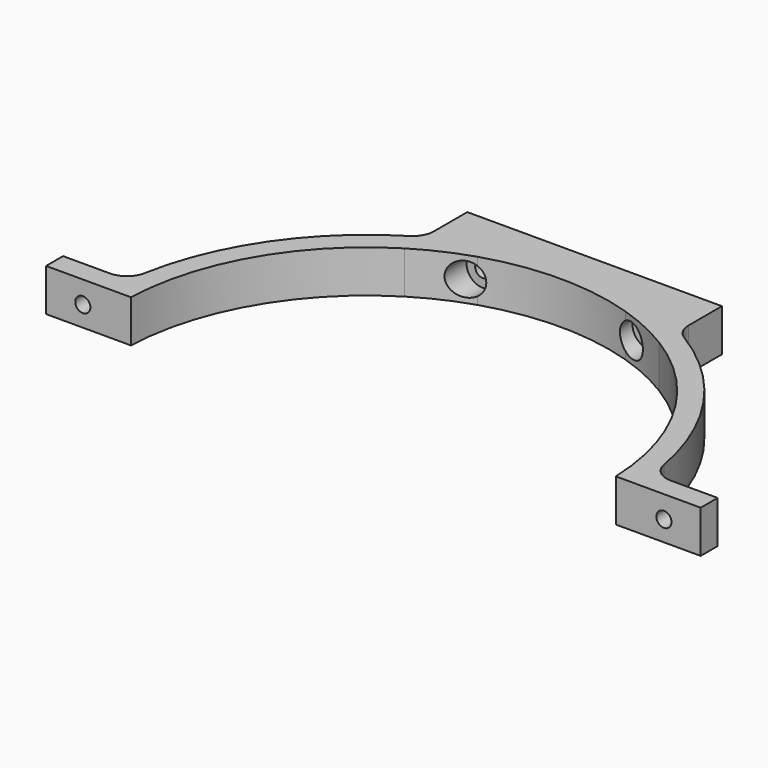
from build123d import *
from build123d import SkipClean  # not in build123d's __all__

# Parameters (mm, degrees)
F1_DEPTH       = 10
F3_D           = 3.556
F3_CBORE_D     = 7.62
F3_CBORE_DEPTH = 10
F4_DEPTH       = 10.0010001
F6_D           = 3.556
F7_R           = 5


with BuildPart() as f1:
    # F0 (on Top) → F1 (new body)
    with BuildSketch(Plane.XY):
        with BuildLine():
            ThreePointArc((30, 48.6428052234), (49.4079280032, 28.7224502859), (57.1149936532, 2))
            Line((57.1149936532, 2), (57.1149936532, 7))
            Line((57.1149936532, 7), (61.7545342465, 7))
            ThreePointArc((61.7545342465, 7), (51.6442091706, 34.5759766187), (30, 54.4299779533))
            Line((30, 54.4299779533), (30, 48.6428052234))
        make_face()
        with BuildLine():
            ThreePointArc((17.4212513902, 54.4299779533), (23.8865362266, 51.9187431194), (30, 48.6428052234))
            Line((30, 48.6428052234), (30, 54.4299779533))
            Line((30, 54.4299779533), (17.4212513902, 54.4299779533))
        make_face()
        with BuildLine():
            ThreePointArc((-17.4212513902, 54.4299779533), (0, 57.15), (17.4212513902, 54.4299779533))
            Line((17.4212513902, 54.4299779533), (30, 54.4299779533))
            ThreePointArc((30, 54.4299779533), (15.4886954339, 60.1890589207), (7.62e-08, 62.15))
            ThreePointArc((7.62e-08, 62.15), (-15.4886953601, 60.1890589397), (-30, 54.4299779533))
            Line((-30, 54.4299779533), (-17.4212513902, 54.4299779533))
        make_face()
        with BuildLine():
            Line((-30, 54.4299779533), (-30, 48.6428052234))
            ThreePointArc((-30, 48.6428052234), (-23.8865362266, 51.9187431194), (-17.4212513902, 54.4299779533))
            Line((-17.4212513902, 54.4299779533), (-30, 54.4299779533))
        make_face()
        with BuildLine():
            ThreePointArc((-57.1149936532, 2), (-49.4079280032, 28.7224502859), (-30, 48.6428052234))
            Line((-30, 48.6428052234), (-30, 54.4299779533))
            ThreePointArc((-30, 54.4299779533), (-51.6442091706, 34.5759766187), (-61.7545342465, 7))
            Line((-61.7545342465, 7), (-57.1149936532, 7))
            Line((-57.1149936532, 7), (-57.1149936532, 2))
        make_face()
        with BuildLine():
            Line((-77.1149936532, 2), (-62.1178114553, 2))
            ThreePointArc((-62.1178114553, 2), (-61.9866074843, 4.5036643506), (-61.7545342465, 7))
            Line((-61.7545342465, 7), (-77.1149936532, 7))
            Line((-77.1149936532, 7), (-77.1149936532, 2))
        make_face()
        with BuildLine():
            Line((-62.1178114553, 2), (-57.1149936532, 2))
            Line((-57.1149936532, 2), (-57.1149936532, 7))
            Line((-57.1149936532, 7), (-61.7545342465, 7))
            ThreePointArc((-61.7545342465, 7), (-61.9866074843, 4.5036643506), (-62.1178114553, 2))
        make_face()
        with BuildLine():
            Line((57.1149936532, 7), (57.1149936532, 2))
            Line((57.1149936532, 2), (62.1178114553, 2))
            ThreePointArc((62.1178114553, 2), (61.9866074843, 4.5036643506), (61.7545342465, 7))
            Line((61.7545342465, 7), (57.1149936532, 7))
        make_face()
        with BuildLine():
            ThreePointArc((61.7545342465, 7), (61.9866074843, 4.5036643506), (62.1178114553, 2))
            Line((62.1178114553, 2), (77.1149936532, 2))
            Line((77.1149936532, 2), (77.1149936532, 7))
            Line((77.1149936532, 7), (61.7545342465, 7))
        make_face()
        with BuildLine():
            Line((-30, 62.15), (-30, 54.4299779533))
            ThreePointArc((-30, 54.4299779533), (-15.4886953601, 60.1890589397), (7.62e-08, 62.15))
            Line((7.62e-08, 62.15), (-30, 62.15))
        make_face()
        with BuildLine():
            ThreePointArc((7.62e-08, 62.15), (15.4886954339, 60.1890589207), (30, 54.4299779533))
            Line((30, 54.4299779533), (30, 62.15))
            Line((30, 62.15), (7.62e-08, 62.15))
        make_face()
        with BuildLine():
            Line((-30, 48.6428052234), (30, 48.6428052234))
            ThreePointArc((30, 48.6428052234), (23.8865362266, 51.9187431194), (17.4212513902, 54.4299779533))
            Line((17.4212513902, 54.4299779533), (-17.4212513902, 54.4299779533))
            ThreePointArc((-17.4212513902, 54.4299779533), (-23.8865362266, 51.9187431194), (-30, 48.6428052234))
        make_face()
        Polygon((-30, 62.15), (7.62e-08, 62.15), (30, 62.15), (30, 67.15), (-30, 67.15), align=None)
    extrude(amount=F1_DEPTH)

    # F3 (through all)
    with Locations(Plane.XZ.offset(-48.6428052234)):
        with Locations((-19.558, 4.9517820589), (19.558, 4.9517820589)):
            CounterBoreHole(F3_D / 2, F3_CBORE_D / 2, F3_CBORE_DEPTH)

    # F0 (on Top) → F4 (cut, through all)
    with BuildSketch(Plane.XY):
        with BuildLine():
            Line((-30, 48.6428052234), (30, 48.6428052234))
            ThreePointArc((30, 48.6428052234), (23.8865362266, 51.9187431194), (17.4212513902, 54.4299779533))
            Line((17.4212513902, 54.4299779533), (-17.4212513902, 54.4299779533))
            ThreePointArc((-17.4212513902, 54.4299779533), (-23.8865362266, 51.9187431194), (-30, 48.6428052234))
        make_face()
    with SkipClean():  # cleaning this boolean's faces spoils the solid; the shape is the same uncleaned
        extrude(amount=F4_DEPTH, mode=Mode.SUBTRACT)

    # F6 (through all)
    with Locations(Plane.XZ.offset(-2)):
        with Locations((-68.453, 4.78035165), (68.453, 4.78035165)):
            Hole(F6_D / 2)

    # F7
    f7_edges = [f1.edges().sort_by_distance(p)[0] for p in [
        (-61.754534, 7, 5),
        (61.754534, 7, 5),
        (30, 54.429978, 5),
        (-30, 54.429978, 5),
    ]]
    fillet(f7_edges, radius=F7_R)


solid = f1.part
